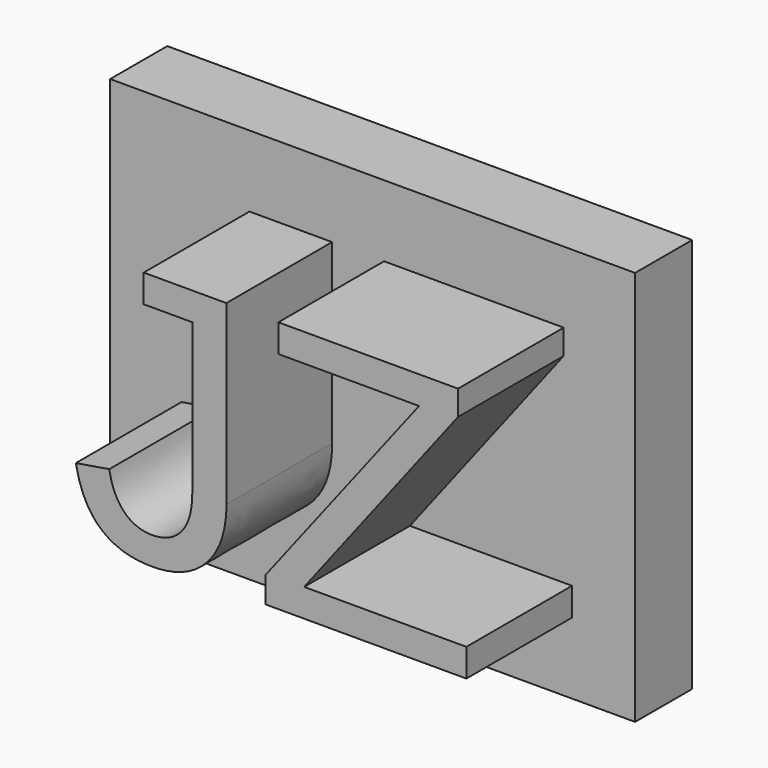
from build123d import *

# Parameters (mm, degrees)
F0_TEXT_SIZE = 35.2777777778
F1_DEPTH     = 12.7
F2_W         = 50.4434739583
F2_H         = 37.9860086806
F3_DEPTH     = 6.858


# Not quite as in the source:
# - Text() gives the source's letters only with a copy of the font that has no kerning and outlines rounded to 1/6400 em; it was checked with that copy


with BuildPart() as f1:
    # F0 (on Front) → F1 (new body)
    with BuildSketch(Plane.XZ):
        with Locations((-18.104821949, -12.1408806597)):
            Text('JZ', F0_TEXT_SIZE, font='Arimo', text_align=(TextAlign.LEFT, TextAlign.BOTTOM))
    extrude(amount=F1_DEPTH)

    # F2 (on Front) → F3 (join)
    with BuildSketch(Plane.XZ):
        with Locations((0.8101303079, -0.0058763194)):
            Rectangle(F2_W, F2_H)
    extrude(amount=-F3_DEPTH)


solid = f1.part
